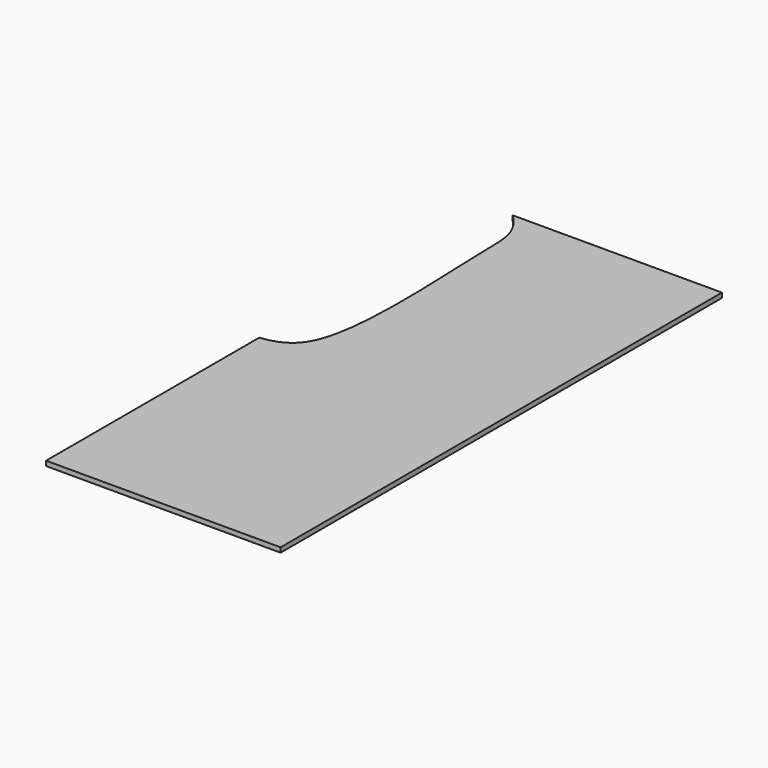
from build123d import *

# Parameters (mm, degrees)
F0_W     = 880
F0_H     = 2070
F1_DEPTH = 9
F3_DEPTH = 25


with BuildPart() as f1:
    # F0 (on Top) → F1 (new body, symmetric)
    with BuildSketch(Plane.XY):
        Rectangle(F0_W, F0_H)
    extrude(amount=F1_DEPTH, both=True)

    # F2 (on face) → F3 (cut)
    with BuildSketch(Plane(origin=(0, 0, -9), x_dir=(1, 0, 0), z_dir=(0, 0, -1))):
        with BuildLine():
            Line((-440, -1035), (-345.1635837555, -1035))
            add(Edge.make_bspline(
                [(-345.1635837555, -1035), (-264.3917672013, -953.7238384219), (-282.7083415362, -828.3101050302), (-218.7463566298, -15.6652863678), (-387.7181019401, 28.374090669), (-440, 35.421974957)],
                knots=[0, 0, 0, 0, 0.2848252576, 0.7699167532, 1, 1, 1, 1], degree=3))
            Line((-440, 35.421974957), (-440, -1035))
        make_face()
    extrude(amount=-F3_DEPTH, mode=Mode.SUBTRACT)


solid = f1.part
